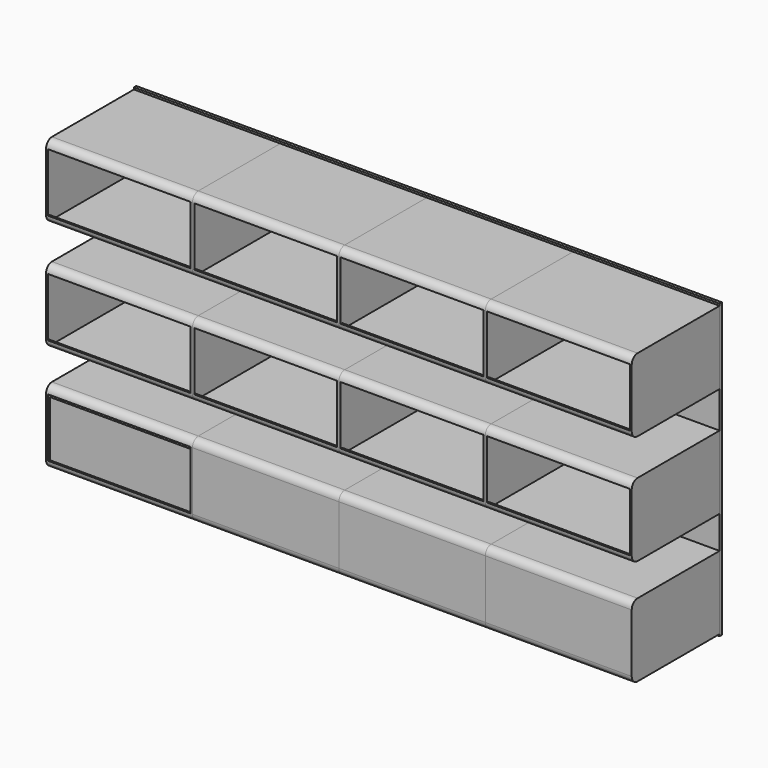
from build123d import *

# Parameters (mm, degrees)
F0_W      = 800
F0_H      = 400
F1_DEPTH  = 4
F4_DEPTH  = 200
F11_T     = -2.5
F13_W     = 8.70706141
F13_H     = 79.0953636169
F14_DEPTH = 200


# Not quite as in the source:
# - a shell that OpenCascade refuses in one call is made with other operations: the cavity is built on its own and cut out


with BuildPart() as f1:
    # F0 (on Front) → F1 (new body)
    with BuildSketch(Plane.XZ):
        Rectangle(F0_W, F0_H)
    extrude(amount=F1_DEPTH)


with BuildPart() as f4:
    # F3 (on offset) → F4 (new body)
    with BuildSketch(Plane.YZ.offset(-400)):
        with BuildLine():
            Line((-144, -197.3634083569), (-4, -197.3634083569))
            Line((-4, -197.3634083569), (-4, -97.3634083569))
            Line((-4, -97.3634083569), (-144, -97.3634083569))
            ThreePointArc((-144, -97.3634083569), (-151.0710678119, -100.292340545), (-154, -107.3634083569))
            Line((-154, -107.3634083569), (-154, -187.3634083569))
            ThreePointArc((-154, -187.3634083569), (-151.0710678119, -194.4344761688), (-144, -197.3634083569))
        make_face()
    extrude(amount=F4_DEPTH)


with BuildPart() as f6_1:
    # F6: instance of F4
    add(f4.part.mirror(Plane.YZ.offset(-200)))


with BuildPart() as f8_1:
    # F8: instance of F6_1
    add(f6_1.part.mirror(Plane.YZ))


with BuildPart() as f10_1:
    # F10: instance of F8_1
    add(f8_1.part.mirror(Plane.YZ.offset(200)))


with BuildPart() as f4_1:
    add(f4.part)

    # F11: a shell. OpenCascade refuses it in one call, so the cavity is built on its own and cut out:
    # the body offset inwards by the wall thickness, plus a prism from it out through each open face.
    f11_core = offset(f4_1.part, amount=F11_T, mode=Mode.PRIVATE)
    f11_exits = [f11_core.faces().sort_by_distance(p)[0] for p in [
        (-300, -151.5, -147.363408),
    ]]
    add(f11_core, mode=Mode.SUBTRACT)
    extrude(f11_exits, amount=-F11_T, mode=Mode.SUBTRACT)


with BuildPart() as f14:
    # F13 (on offset) → F14 (new body)
    with BuildSketch(Plane.YZ.offset(-400)):
        with Locations((-146.2915912271, -151.602640748)):
            Rectangle(F13_W, F13_H)
    extrude(amount=F14_DEPTH)


with BuildPart() as f15_1:
    # F15: instance of F4
    add(f4_1.part.mirror(Plane.XY))


with BuildPart() as f17_1:
    # F17: instance of F15_1
    add(f15_1.part.mirror(Plane.YZ.offset(-200)))


with BuildPart() as f19_1:
    # F19: instance of F17_1
    add(f17_1.part.mirror(Plane.YZ))


with BuildPart() as f21_1:
    # F21: instance of F19_1
    add(f19_1.part.mirror(Plane.YZ.offset(200)))


with BuildPart() as f22_1:
    # F22: copy of F15_1
    add(f15_1.part.moved(Location((0, 0, -150))))


with BuildPart() as f23_1:
    # F23: copy of F22_1
    add(f22_1.part.moved(Location((200, 0, 0))))


with BuildPart() as f24_1:
    # F24: copy of F23_1
    add(f23_1.part.moved(Location((200, 0, 0))))


with BuildPart() as f25_1:
    # F25: copy of F24_1
    add(f24_1.part.moved(Location((200, 0, 0))))


solid = Compound([f1.part, f6_1.part, f8_1.part, f10_1.part, f4_1.part, f14.part, f15_1.part, f17_1.part, f19_1.part, f21_1.part, f22_1.part, f23_1.part, f24_1.part, f25_1.part])
